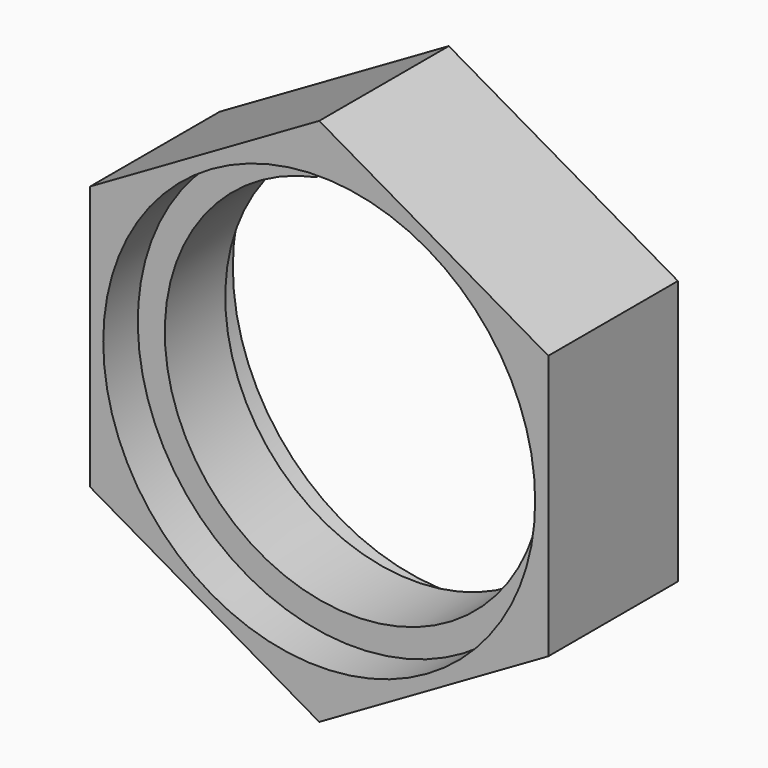
from build123d import *
from build123d import SkipClean  # not in build123d's __all__

# Parameters (mm, degrees)
F0_R     = 44.45
F1_DEPTH = 38.1
F2_R     = 50.8
F3_DEPTH = 10.16
F4_R     = 50.8
F5_DEPTH = 10.16
F7_DEPTH = 25.4
F8_SCALE = 0.75


with BuildPart() as f1:
    # F0 (on Front) → F1 (new body)
    with BuildSketch(Plane.XZ):
        Polygon((53.8927608775, 31.115), (0, 62.23), (-53.8927608775, 31.115), (-53.8927608775, -31.115), (0, -62.23), (53.8927608775, -31.115), align=None)
        Circle(F0_R, mode=Mode.SUBTRACT)
    extrude(amount=F1_DEPTH)

    # F2 (on face) → F3 (cut)
    with BuildSketch(Plane.XZ.offset(38.1)):
        Circle(F2_R)
    extrude(amount=-F3_DEPTH, mode=Mode.SUBTRACT)

    # F4 (on face) → F5 (cut)
    with BuildSketch(Plane(origin=(0, 0, 0), x_dir=(-1, 0, 0), z_dir=(0, 1, 0))):
        Circle(F4_R)
    extrude(amount=-F5_DEPTH, mode=Mode.SUBTRACT)

    # F6 (on face) → F7 (cut)
    with BuildSketch(Plane(origin=(0, -10.16, 0), x_dir=(-1, 0, 0), z_dir=(0, 1, 0))):
        with BuildLine():
            Line((7.7186614973, 43.7747046214), (8.8213274255, 50.028233853))
            ThreePointArc((8.8213274255, 50.028233853), (0, 50.8), (-8.8213274255, 50.028233853))
            Line((-8.8213274255, 50.028233853), (-7.7186614973, 43.7747046214))
            ThreePointArc((-7.7186614973, 43.7747046214), (0, 44.45), (7.7186614973, 43.7747046214))
        make_face()
        with BuildLine():
            Line((-7.7186614973, 43.7747046214), (-8.8213274255, 50.028233853))
            Line((-8.8213274255, 50.028233853), (-8.8213274255, 43.5658889781))
            ThreePointArc((-8.8213274255, 43.5658889781), (-8.2706535041, 43.6737769218), (-7.7186614973, 43.7747046214))
        make_face()
        with BuildLine():
            Line((8.8213274255, 43.5658889781), (8.8213274255, 50.028233853))
            Line((8.8213274255, 50.028233853), (7.7186614973, 43.7747046214))
            ThreePointArc((7.7186614973, 43.7747046214), (8.2706535041, 43.6737769218), (8.8213274255, 43.5658889781))
        make_face()
    with SkipClean():  # cleaning this boolean's faces spoils the solid; the shape is the same uncleaned
        extrude(amount=-F7_DEPTH, mode=Mode.SUBTRACT)


with BuildPart() as f1_1:
    # F8: moved
    add(f1.part.scale(F8_SCALE), clean=False)


solid = f1_1.part
